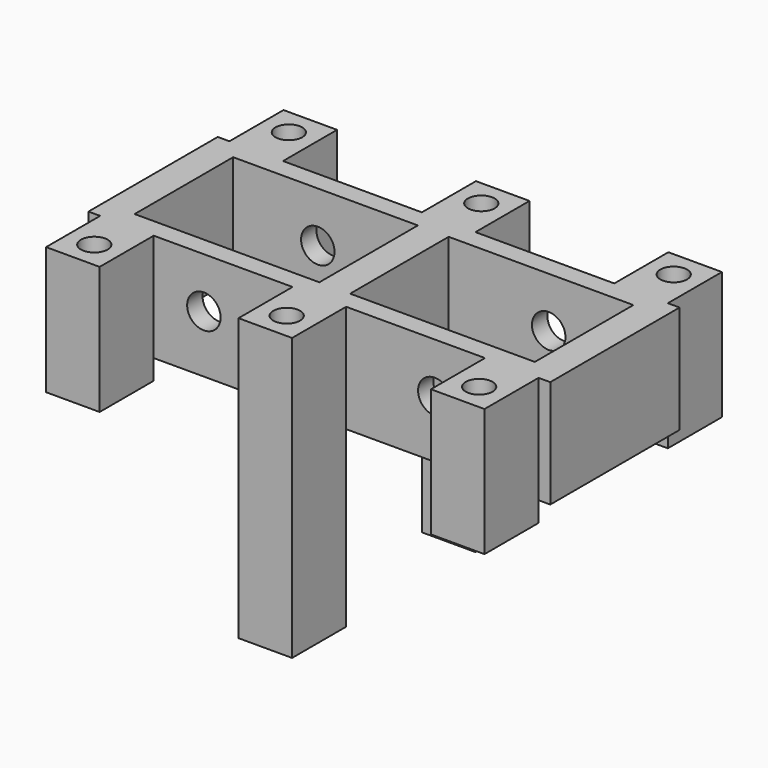
from build123d import *

# Parameters (mm, degrees)
F1_R          = 1.25
F2_DEPTH      = 12.0689655172
F3_W          = 13.7931034483
F3_H          = 9.1954022989
F4_DEPTH      = 8.0469770115
F5_W          = 4
F5_H          = 5.0459770115
F5_R          = 1
F6_DEPTH      = 8.0459770115
F6_DEPTH_BACK = 1.4942528736
F7_W          = 4
F7_H          = 5.0459770115
F7_R          = 1
F8_DEPTH      = 12.9885057471
F8_DEPTH_BACK = 8.0459770115


with BuildPart() as f2:
    # F1 (on Front) → F2 (new body)
    with BuildSketch(Plane.XZ):
        Polygon((-17.2413793103, 0), (0, 0), (17.2413793103, 0), (17.2413793103, 1.724137931), (17.2413793103, 8.0459770115), (0, 8.0459770115), (-17.2413793103, 8.0459770115), (-17.2413793103, 1.724137931), align=None)
        with Locations((-8.6206896552, 4.2873563218)):
            Circle(F1_R, mode=Mode.SUBTRACT)
        with Locations((8.6206896552, 4.2873563218)):
            Circle(F1_R, mode=Mode.SUBTRACT)
    extrude(amount=F2_DEPTH)

    # F3 (on face) → F4 (cut, through all)
    with BuildSketch(Plane.XY.offset(8.0459770115)):
        with Locations((-8.0459770115, -6.0344827586)):
            Rectangle(F3_W, F3_H)
        with Locations((8.0459770115, -6.0344827586)):
            Rectangle(F3_W, F3_H)
    extrude(amount=-F4_DEPTH, mode=Mode.SUBTRACT)

    # F5 (on face) → F6 (join, two sides)
    with BuildSketch(Plane(origin=(0, 0, 0), x_dir=(1, 0, 0), z_dir=(0, 0, -1))) as f6_sk:
        with Locations((-14.367816092, 14.591954023)):
            Rectangle(F5_W, F5_H)
        with Locations((-14.367816092, 15.1149425287)):
            Circle(F5_R, mode=Mode.SUBTRACT)
        with Locations((14.367816092, 14.591954023)):
            Rectangle(F5_W, F5_H)
        with Locations((14.367816092, 15.1149425287)):
            Circle(F5_R, mode=Mode.SUBTRACT)
        with Locations((-14.367816092, -2.5229885057)):
            Rectangle(F5_W, F5_H)
        with Locations((-14.367816092, -3.0459770115)):
            Circle(F5_R, mode=Mode.SUBTRACT)
        with Locations((14.367816092, -2.5229885057)):
            Rectangle(F5_W, F5_H)
        with Locations((14.367816092, -3.0459770115)):
            Circle(F5_R, mode=Mode.SUBTRACT)
    extrude(amount=-F6_DEPTH)
    extrude(f6_sk.sketch, amount=F6_DEPTH_BACK)

    # F7 (on face) → F8 (join, two sides)
    with BuildSketch(Plane(origin=(0, 0, 0), x_dir=(1, 0, 0), z_dir=(0, 0, -1))) as f8_sk:
        with Locations((0, 14.591954023)):
            Rectangle(F7_W, F7_H)
        with Locations((0, 15.1149425287)):
            Circle(F7_R, mode=Mode.SUBTRACT)
        with Locations((0, -2.5229885057)):
            Rectangle(F7_W, F7_H)
        with Locations((0, -3.0459770115)):
            Circle(F7_R, mode=Mode.SUBTRACT)
    extrude(amount=F8_DEPTH)
    extrude(f8_sk.sketch, amount=-F8_DEPTH_BACK)


solid = f2.part
